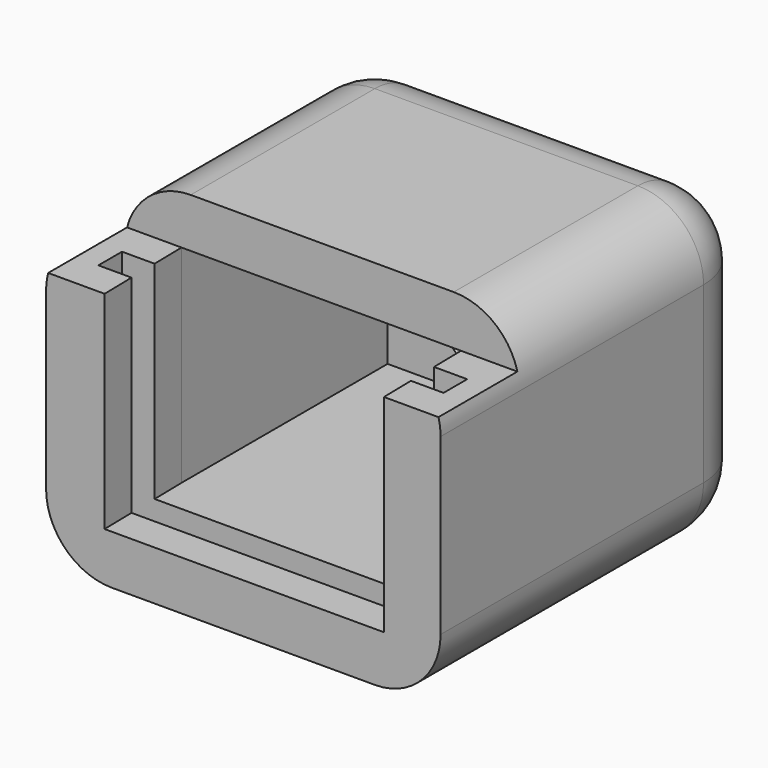
from build123d import *

# Parameters (mm, degrees)
F0_W         = 8.5
F0_H         = 7.834737435
F0_W_2       = 1.7211329822
F0_H_2       = 1.165262565
F0_W_3       = 1.7788670178
F1_DEPTH     = 0.9
F2_DEPTH     = 1.5
F3_DEPTH     = 7.8
F5_W         = 12
F5_H         = 9
F6_DEPTH     = 1.5
F7_R         = 3
F8_DEPTH     = 10.501
F9_T1_DEPTH  = 5.3
F9_T3_DEPTH  = 8
F9_T5_DEPTH  = 12
F9_T7_DEPTH  = 15
F9_S11_W     = 2
F9_S11_H     = 2
F9_T12_DEPTH = 2
F9_S17_W     = 2
F9_S17_H     = 2
F9_T18_DEPTH = 2
F9_S23_W     = 2
F9_S23_H     = 2
F9_T24_DEPTH = 2
F9_S29_W     = 2
F9_S29_H     = 2
F9_T30_DEPTH = 2


# Not quite as in the source:
# - a fillet or chamfer that OpenCascade refuses, or shapes differently, is made with other operations: its cross-section is extruded or revolved along the edge and cut away or added
# - a feature names something its author has since deleted; it is built from what else it names


with BuildPart() as f1:
    # F0 (on Top) → F1 (new body)
    with BuildSketch(Plane.XY):
        with Locations((-0.0288670178, 5.4173687175)):
            Rectangle(F0_W, F0_H)
        Polygon((-6, 1.5), (-6, -1.5), (-4.2211329822, -1.5), (-4.2413398946, -0.45), (-5.25, -0.45), (-5.25, 0.45), (-4.2586601054, 0.45), (-4.2788670178, 1.5), align=None)
        Polygon((4.2211329822, 1.5), (-4.2788670178, 1.5), (-4.2586601054, 0.45), (4.2413398946, 0.45), align=None)
        with Locations((-5.1394335089, 5.4173687175)):
            Rectangle(F0_W_2, F0_H)
        Polygon((4.2586601054, -0.45), (4.2788670178, -1.5), (6, -1.5), (6, 1.5), (4.2211329822, 1.5), (4.2413398946, 0.45), (5.25, 0.45), (5.25, -0.45), align=None)
        Polygon((-4.2413398946, -0.45), (-4.2211329822, -1.5), (4.2788670178, -1.5), (4.2586601054, -0.45), align=None)
        Polygon((-4.2586601054, 0.45), (-4.2413398946, -0.45), (4.2586601054, -0.45), (4.2413398946, 0.45), align=None)
        Polygon((-5.25, -0.45), (-4.2413398946, -0.45), (-4.2586601054, 0.45), (-5.25, 0.45), align=None)
        Polygon((4.2413398946, 0.45), (4.2586601054, -0.45), (5.25, -0.45), (5.25, 0.45), align=None)
        with Locations((-5.1394335089, 9.9173687175)):
            Rectangle(F0_W_2, F0_H_2)
        with Locations((-0.0288670178, 9.9173687175)):
            Rectangle(F0_W, F0_H_2)
        with Locations((5.1105664911, 9.9173687175)):
            Rectangle(F0_W_3, F0_H_2)
        with Locations((5.1105664911, 5.4173687175)):
            Rectangle(F0_W_3, F0_H)
    extrude(amount=F1_DEPTH)

    # F0 (on Top) → F2 (join)
    with BuildSketch(Plane.XY):
        Polygon((-4.2413398946, -0.45), (-4.2211329822, -1.5), (4.2788670178, -1.5), (4.2586601054, -0.45), align=None)
        Polygon((-6, 1.5), (-6, -1.5), (-4.2211329822, -1.5), (-4.2413398946, -0.45), (-5.25, -0.45), (-5.25, 0.45), (-4.2586601054, 0.45), (-4.2788670178, 1.5), align=None)
        Polygon((4.2586601054, -0.45), (4.2788670178, -1.5), (6, -1.5), (6, 1.5), (4.2211329822, 1.5), (4.2413398946, 0.45), (5.25, 0.45), (5.25, -0.45), align=None)
        Polygon((4.2211329822, 1.5), (-4.2788670178, 1.5), (-4.2586601054, 0.45), (4.2413398946, 0.45), align=None)
        with Locations((-5.1394335089, 5.4173687175)):
            Rectangle(F0_W_2, F0_H)
        with Locations((5.1105664911, 5.4173687175)):
            Rectangle(F0_W_3, F0_H)
        with Locations((-0.0288670178, 5.4173687175)):
            Rectangle(F0_W, F0_H)
        with Locations((-5.1394335089, 9.9173687175)):
            Rectangle(F0_W_2, F0_H_2)
        with Locations((-0.0288670178, 9.9173687175)):
            Rectangle(F0_W, F0_H_2)
        with Locations((5.1105664911, 9.9173687175)):
            Rectangle(F0_W_3, F0_H_2)
    extrude(amount=F2_DEPTH)

    # F0 (on Top) → F3 (join)
    with BuildSketch(Plane.XY):
        Polygon((-6, 1.5), (-6, -1.5), (-4.2211329822, -1.5), (-4.2413398946, -0.45), (-5.25, -0.45), (-5.25, 0.45), (-4.2586601054, 0.45), (-4.2788670178, 1.5), align=None)
        Polygon((4.2586601054, -0.45), (4.2788670178, -1.5), (6, -1.5), (6, 1.5), (4.2211329822, 1.5), (4.2413398946, 0.45), (5.25, 0.45), (5.25, -0.45), align=None)
        with Locations((-5.1394335089, 5.4173687175)):
            Rectangle(F0_W_2, F0_H)
        with Locations((5.1105664911, 5.4173687175)):
            Rectangle(F0_W_3, F0_H)
        with Locations((-5.1394335089, 9.9173687175)):
            Rectangle(F0_W_2, F0_H_2)
        with Locations((-0.0288670178, 9.9173687175)):
            Rectangle(F0_W, F0_H_2)
        with Locations((5.1105664911, 9.9173687175)):
            Rectangle(F0_W_3, F0_H_2)
    extrude(amount=F3_DEPTH)

    # F5 (on offset) → F6 (join)
    with BuildSketch(Plane.XY.offset(7.8)):
        with Locations((0, 6)):
            Rectangle(F5_W, F5_H)
    extrude(amount=F6_DEPTH)

    # F7 (on Front) → F8 (cut, through all)
    with BuildSketch(Plane.XZ):
        with Locations((0, 4.5)):
            Circle(F7_R)
    extrude(amount=-F8_DEPTH, mode=Mode.SUBTRACT)

    # F9: fillet of radius 2 on 8 edges, made by hand

    # F9_s2 → F9_t1 (cut)
    with BuildSketch(Plane.XY.offset(2)):
        with BuildLine():
            ThreePointArc((4, 10.5), (5.4142135624, 9.9142135624), (6, 8.5))
            Line((6, 8.5), (6, 10.5))
            Line((6, 10.5), (4, 10.5))
        make_face()
        with BuildLine():
            ThreePointArc((-4, 10.5), (-5.4142135624, 9.9142135624), (-6, 8.5))
            Line((-6, 8.5), (-6, 10.5))
            Line((-6, 10.5), (-4, 10.5))
        make_face()
    extrude(amount=F9_T1_DEPTH, mode=Mode.SUBTRACT)

    # F9_s4 → F9_t3 (cut)
    with BuildSketch(Plane.YZ.offset(-4)):
        with BuildLine():
            ThreePointArc((10.5, 7.3), (9.9142135624, 8.7142135624), (8.5, 9.3))
            Line((8.5, 9.3), (10.5, 9.3))
            Line((10.5, 9.3), (10.5, 7.3))
        make_face()
        with BuildLine():
            ThreePointArc((8.5, 0), (9.9142135624, 0.5857864376), (10.5, 2))
            Line((10.5, 2), (10.5, 0))
            Line((10.5, 0), (8.5, 0))
        make_face()
    extrude(amount=F9_T3_DEPTH, mode=Mode.SUBTRACT)

    # F9_s6 → F9_t5 (cut)
    with BuildSketch(Plane.XZ.offset(-8.5)):
        with BuildLine():
            ThreePointArc((4, 9.3), (5.4142135624, 8.7142135624), (6, 7.3))
            Line((6, 7.3), (6, 9.3))
            Line((6, 9.3), (4, 9.3))
        make_face()
        with BuildLine():
            ThreePointArc((-4, 9.3), (-5.4142135624, 8.7142135624), (-6, 7.3))
            Line((-6, 7.3), (-6, 9.3))
            Line((-6, 9.3), (-4, 9.3))
        make_face()
    extrude(amount=F9_T5_DEPTH, mode=Mode.SUBTRACT)

    # F9_s8 → F9_t7 (cut)
    with BuildSketch(Plane.XZ.offset(-8.5)):
        with BuildLine():
            ThreePointArc((4, 0), (5.4142135624, 0.5857864376), (6, 2))
            Line((6, 2), (6, 0))
            Line((6, 0), (4, 0))
        make_face()
        with BuildLine():
            ThreePointArc((-4, 0), (-5.4142135624, 0.5857864376), (-6, 2))
            Line((-6, 2), (-6, 0))
            Line((-6, 0), (-4, 0))
        make_face()
    extrude(amount=F9_T7_DEPTH, mode=Mode.SUBTRACT)


with BuildPart() as f9_tool10:
    # F9_s11 → F9_t12 (new body)
    with BuildSketch(Plane.XY.offset(2)):
        with Locations((5, 9.5)):
            Rectangle(F9_S11_W, F9_S11_H)
    extrude(amount=-F9_T12_DEPTH)

    # F9_s13 → F9_t14 (revolve, cut)
    with BuildSketch(Plane(origin=(4, 8.5, 2), x_dir=(-0.7071067812, -0.7071067812, 0), z_dir=(0.7071067812, -0.7071067812, 0))):
        with BuildLine():
            ThreePointArc((0, -2), (2, 0), (0, 2))
            Line((0, 2), (0, -2))
        make_face()
    revolve(axis=Axis((4, 8.5, 2), (0, 0, -1)), mode=Mode.SUBTRACT)


with BuildPart() as f1_1:
    add(f1.part)

    # F9_t9: cut F9_tool10
    add(f9_tool10.part, mode=Mode.SUBTRACT)


with BuildPart() as f9_tool16:
    # F9_s17 → F9_t18 (new body)
    with BuildSketch(Plane.XY.offset(7.3)):
        with Locations((5, 9.5)):
            Rectangle(F9_S17_W, F9_S17_H)
    extrude(amount=F9_T18_DEPTH)

    # F9_s19 → F9_t20 (revolve, cut)
    with BuildSketch(Plane(origin=(4, 8.5, 7.3), x_dir=(-0.7071067812, -0.7071067812, 0), z_dir=(-0.7071067812, 0.7071067812, 0))):
        with BuildLine():
            ThreePointArc((0, -2), (2, 0), (0, 2))
            Line((0, 2), (0, -2))
        make_face()
    revolve(axis=Axis((4, 8.5, 7.3), (0, 0, 1)), mode=Mode.SUBTRACT)


with BuildPart() as f1_2:
    add(f1_1.part)

    # F9_t15: cut F9_tool16
    add(f9_tool16.part, mode=Mode.SUBTRACT)


with BuildPart() as f9_tool22:
    # F9_s23 → F9_t24 (new body)
    with BuildSketch(Plane.YZ.offset(-4)):
        with Locations((9.5, 8.3)):
            Rectangle(F9_S23_W, F9_S23_H)
    extrude(amount=-F9_T24_DEPTH)

    # F9_s25 → F9_t26 (revolve, cut)
    with BuildSketch(Plane(origin=(-4, 8.5, 7.3), x_dir=(0, -0.7071067812, -0.7071067812), z_dir=(0, 0.7071067812, -0.7071067812))):
        with BuildLine():
            ThreePointArc((0, -2), (2, 0), (0, 2))
            Line((0, 2), (0, -2))
        make_face()
    revolve(axis=Axis((-4, 8.5, 7.3), (-1, 0, 0)), mode=Mode.SUBTRACT)


with BuildPart() as f1_3:
    add(f1_2.part)

    # F9_t21: cut F9_tool22
    add(f9_tool22.part, mode=Mode.SUBTRACT)


with BuildPart() as f9_tool28:
    # F9_s29 → F9_t30 (new body)
    with BuildSketch(Plane.YZ.offset(-4)):
        with Locations((9.5, 1)):
            Rectangle(F9_S29_W, F9_S29_H)
    extrude(amount=-F9_T30_DEPTH)

    # F9_s31 → F9_t32 (revolve, cut)
    with BuildSketch(Plane(origin=(-4, 8.5, 2), x_dir=(0, -0.7071067812, 0.7071067812), z_dir=(0, -0.7071067812, -0.7071067812))):
        with BuildLine():
            ThreePointArc((0, -2), (2, 0), (0, 2))
            Line((0, 2), (0, -2))
        make_face()
    revolve(axis=Axis((-4, 8.5, 2), (-1, 0, 0)), mode=Mode.SUBTRACT)


with BuildPart() as f1_4:
    add(f1_3.part)

    # F9_t27: cut F9_tool28
    add(f9_tool28.part, mode=Mode.SUBTRACT)


solid = f1_4.part
